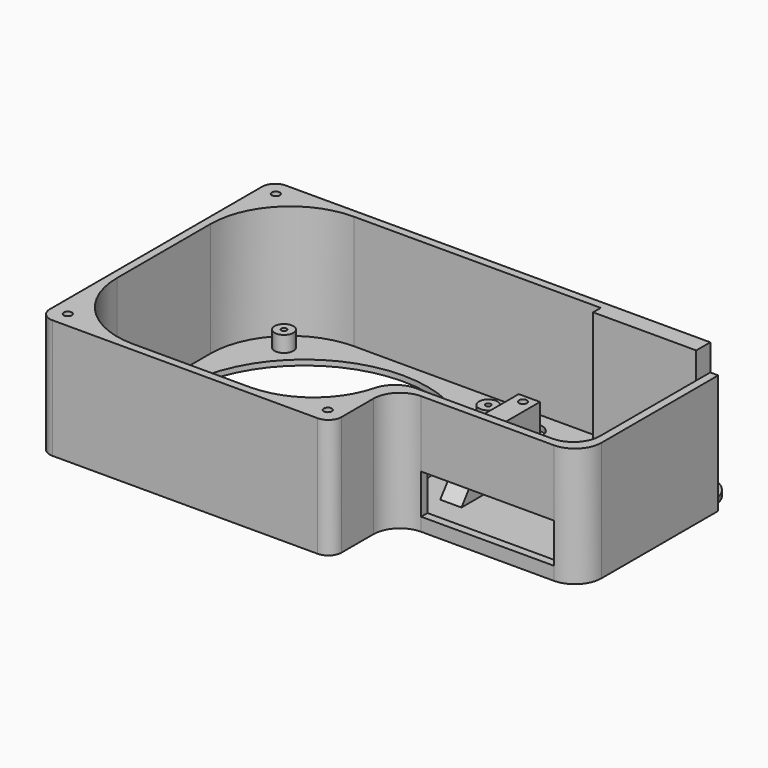
from build123d import *

# Parameters (mm, degrees)
F0_R        = 3.5
F0_R_2      = 46.5
F0_W        = 8
F0_H        = 37
F0_R_3      = 5
F1_DEPTH    = 2
F0_R_4      = 1.5
F2_DEPTH    = 22
F0_W_2      = 38.8732933998
F0_H_2      = 3.6201002002
F0_W_3      = 3
F0_H_3      = 27
F3_DEPTH    = 45
F4_R        = 29.99999
F5_R        = 10
F6_W        = 50
F6_H        = 15
F7_DEPTH    = 5
F8_R        = 5
F0_R_5      = 1
F9_DEPTH    = 8
F10_R       = 1.5
F11_DEPTH   = 25
F12_SIZE2   = 19.99999
F12_SIZE    = 14.99999
F12_2_SIZE2 = 19.99999
F12_2_SIZE  = 14.99999


# Not quite as in the source:
# - a fillet or chamfer is up to 0.001 mm smaller than in the source, because OpenCascade refuses the exact size


with BuildPart() as f1:
    # F0 (on Top) → F1 (new body)
    with BuildSketch(Plane.XY):
        Polygon((126.1267066002, 107), (3, 107), (3, 3), (107, 3), (107, 30), (107, 33), (177, 33), (177, 95), (177, 107), (165, 107), (165, 103.3798997998), (126.1267066002, 103.3798997998), align=None)
        with Locations((17.5, 16.5)):
            Circle(F0_R, mode=Mode.SUBTRACT)
        with Locations((94.5, 16.5)):
            Circle(F0_R, mode=Mode.SUBTRACT)
        with Locations((56, 55)):
            Circle(F0_R_2, mode=Mode.SUBTRACT)
        with Locations((17.5, 93.5)):
            Circle(F0_R, mode=Mode.SUBTRACT)
        with Locations((118, 65)):
            Rectangle(F0_W, F0_H, mode=Mode.SUBTRACT)
        with Locations((171, 65)):
            Rectangle(F0_W, F0_H, mode=Mode.SUBTRACT)
        with Locations((94.5, 93.5)):
            Circle(F0_R, mode=Mode.SUBTRACT)
        with Locations((107, 97)):
            Circle(F0_R_3, mode=Mode.SUBTRACT)
    extrude(amount=F1_DEPTH)

    # F0 (on Top) → F2 (join)
    with BuildSketch(Plane.XY):
        with Locations((118, 65)):
            Rectangle(F0_W, F0_H)
        with Locations((118, 65.5)):
            Circle(F0_R_4, mode=Mode.SUBTRACT)
        with Locations((118, 80.5)):
            Circle(F0_R_4, mode=Mode.SUBTRACT)
        with Locations((171, 65)):
            Rectangle(F0_W, F0_H)
        with Locations((171, 65.5)):
            Circle(F0_R_4, mode=Mode.SUBTRACT)
        with Locations((171, 80.5)):
            Circle(F0_R_4, mode=Mode.SUBTRACT)
    extrude(amount=F2_DEPTH)

    # F0 (on Top) → F3 (join)
    with BuildSketch(Plane.XY):
        Polygon((3, 110), (0, 110), (0, 3), (3, 3), (3, 107), align=None)
        Polygon((165, 110), (3, 110), (3, 107), (126.1267066002, 107), (165, 107), align=None)
        Polygon((3, 3), (0, 3), (0, 0), (110, 0), (110, 3), (107, 3), align=None)
        with Locations((145.5633533001, 105.1899498999)):
            Rectangle(F0_W_2, F0_H_2)
        with Locations((108.5, 16.5)):
            Rectangle(F0_W_3, F0_H_3)
        Polygon((107, 33), (107, 30), (110, 30), (177, 30), (177, 33), align=None)
        Polygon((180, 30), (180, 95), (177, 95), (177, 33), (177, 30), align=None)
    extrude(amount=F3_DEPTH)

    # F4 (radius 30 in the source; OpenCascade refuses exactly that, so slightly less here)
    f4_edges = [f1.edges().sort_by_distance(p)[0] for p in [
        (3, 107, 23.5),
        (3, 3, 23.5),
        (107, 3, 23.5),
    ]]
    fillet(f4_edges, radius=F4_R)

    # F5
    f5_edges = [f1.edges().sort_by_distance(p)[0] for p in [
        (177, 33, 23.5),
        (180, 30, 22.5),
        (110, 30, 22.5),
        (107, 33, 23.5),
        (177, 107, 1),
    ]]
    fillet(f5_edges, radius=F5_R)

    # F6 (on face) → F7 (cut)
    with BuildSketch(Plane.XZ.offset(-30)):
        with Locations((145, 12.5)):
            Rectangle(F6_W, F6_H)
    extrude(amount=-F7_DEPTH, mode=Mode.SUBTRACT)

    # F8
    f8_edges = [f1.edges().sort_by_distance(p)[0] for p in [
        (110, 0, 22.5),
        (0, 0, 22.5),
        (0, 110, 22.5),
    ]]
    fillet(f8_edges, radius=F8_R)

    # F0 (on Top) → F9 (join)
    with BuildSketch(Plane.XY):
        with Locations((94.5, 93.5)):
            Circle(F0_R)
        with Locations((94.5, 93.5)):
            Circle(F0_R_5, mode=Mode.SUBTRACT)
        with Locations((17.5, 93.5)):
            Circle(F0_R)
        with Locations((17.5, 93.5)):
            Circle(F0_R_5, mode=Mode.SUBTRACT)
        with Locations((17.5, 16.5)):
            Circle(F0_R)
        with Locations((17.5, 16.5)):
            Circle(F0_R_5, mode=Mode.SUBTRACT)
        with Locations((94.5, 16.5)):
            Circle(F0_R)
        with Locations((94.5, 16.5)):
            Circle(F0_R_5, mode=Mode.SUBTRACT)
    extrude(amount=F9_DEPTH)

    # F10 (on face) → F11 (cut)
    with BuildSketch(Plane.XY.offset(45)):
        with Locations((6, 104)):
            Circle(F10_R)
        with Locations((6, 6)):
            Circle(F10_R)
        with Locations((104, 6)):
            Circle(F10_R)
    extrude(amount=-F11_DEPTH, mode=Mode.SUBTRACT)

    # F12 (size 15 and 20 in the source; OpenCascade refuses exactly that, so slightly less here)
    f12_edges = [f1.edges().sort_by_distance(p)[0] for p in [
        (118, 46.5, 22),
    ]]
    f12_side = f1.faces().sort_by_distance((118, 83.12145, 22))[0]
    chamfer(f12_edges, length=F12_SIZE, length2=F12_SIZE2, reference=f12_side)

    # F12#2 (size 15 and 20 in the source; OpenCascade refuses exactly that, so slightly less here)
    f12_2_edges = [f1.edges().sort_by_distance(p)[0] for p in [
        (171, 46.5, 22),
    ]]
    f12_2_side = f1.faces().sort_by_distance((171, 83.12145, 22))[0]
    chamfer(f12_2_edges, length=F12_2_SIZE, length2=F12_2_SIZE2, reference=f12_2_side)


solid = f1.part
